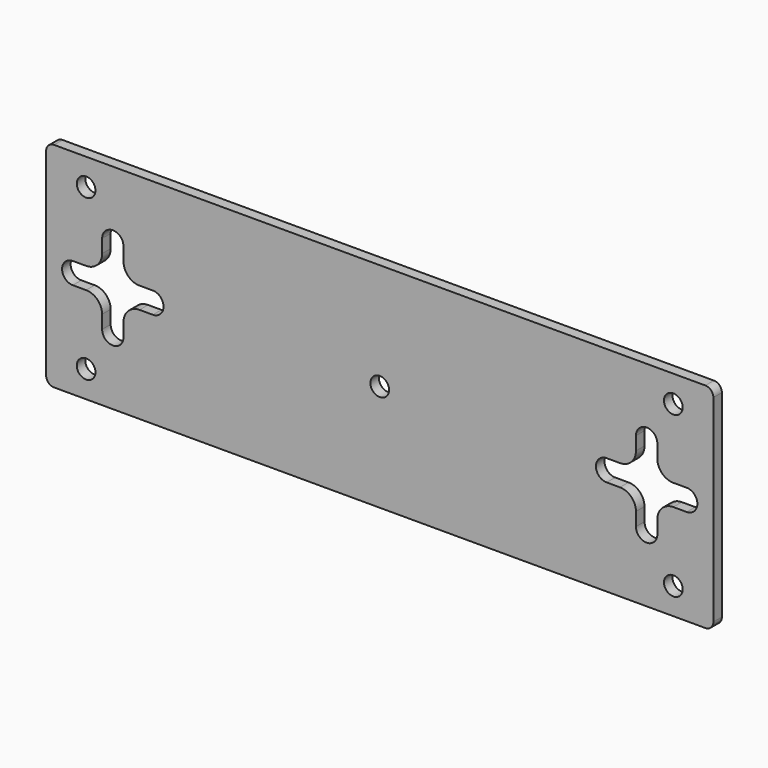
from build123d import *

# Parameters (mm, degrees)
F0_W     = 125
F0_H     = 40
F0_R     = 1.75
F1_DEPTH = 2
F2_R     = 1.5
F3_R     = 3


# Not quite as in the source:
# - a feature names something its author has since deleted; it is built from what else it names


with BuildPart() as f1:
    # F0 (on Front) → F1 (new body)
    with BuildSketch(Plane.XZ):
        Rectangle(F0_W, F0_H)
        with Locations((-55, -15)):
            Circle(F0_R, mode=Mode.SUBTRACT)
        with Locations((55, -15)):
            Circle(F0_R, mode=Mode.SUBTRACT)
        with BuildLine():
            Line((-57.5, 2), (-52, 2))
            Line((-52, 2), (-52, 7.5))
            ThreePointArc((-52, 7.5), (-50, 9.5), (-48, 7.5))
            Line((-48, 7.5), (-48, 2))
            Line((-48, 2), (-42.5, 2))
            ThreePointArc((-42.5, 2), (-40.5, 0), (-42.5, -2))
            Line((-42.5, -2), (-48, -2))
            Line((-48, -2), (-48, -7.5))
            ThreePointArc((-48, -7.5), (-50, -9.5), (-52, -7.5))
            Line((-52, -7.5), (-52, -2))
            Line((-52, -2), (-57.5, -2))
            ThreePointArc((-57.5, -2), (-59.5, 0), (-57.5, 2))
        make_face(mode=Mode.SUBTRACT)
        with Locations((-55, 15)):
            Circle(F0_R, mode=Mode.SUBTRACT)
        Circle(F0_R, mode=Mode.SUBTRACT)
        with BuildLine():
            Line((42.5, 2), (48, 2))
            Line((48, 2), (48, 7.5))
            ThreePointArc((48, 7.5), (50, 9.5), (52, 7.5))
            Line((52, 7.5), (52, 2))
            Line((52, 2), (57.5, 2))
            ThreePointArc((57.5, 2), (59.5, 0), (57.5, -2))
            Line((57.5, -2), (52, -2))
            Line((52, -2), (52, -7.5))
            ThreePointArc((52, -7.5), (50, -9.5), (48, -7.5))
            Line((48, -7.5), (48, -2))
            Line((48, -2), (42.5, -2))
            ThreePointArc((42.5, -2), (40.5, 0), (42.5, 2))
        make_face(mode=Mode.SUBTRACT)
        with Locations((55, 15)):
            Circle(F0_R, mode=Mode.SUBTRACT)
    extrude(amount=F1_DEPTH)

    # F2
    f2_edges = [f1.edges().sort_by_distance(p)[0] for p in [
        (-62.5, -1, 20),
        (62.5, -1, 20),
        (-62.5, -1, -20),
        (62.5, -1, -20),
    ]]
    fillet(f2_edges, radius=F2_R)

    # F3
    f3_edges = [f1.edges().sort_by_distance(p)[0] for p in [
        (-48, -1, 2),
        (-52, -1, 2),
        (-52, -1, -2),
        (-48, -1, -2),
        (52, -1, 2),
        (48, -1, 2),
        (48, -1, -2),
        (52, -1, -2),
    ]]
    fillet(f3_edges, radius=F3_R)


solid = f1.part
